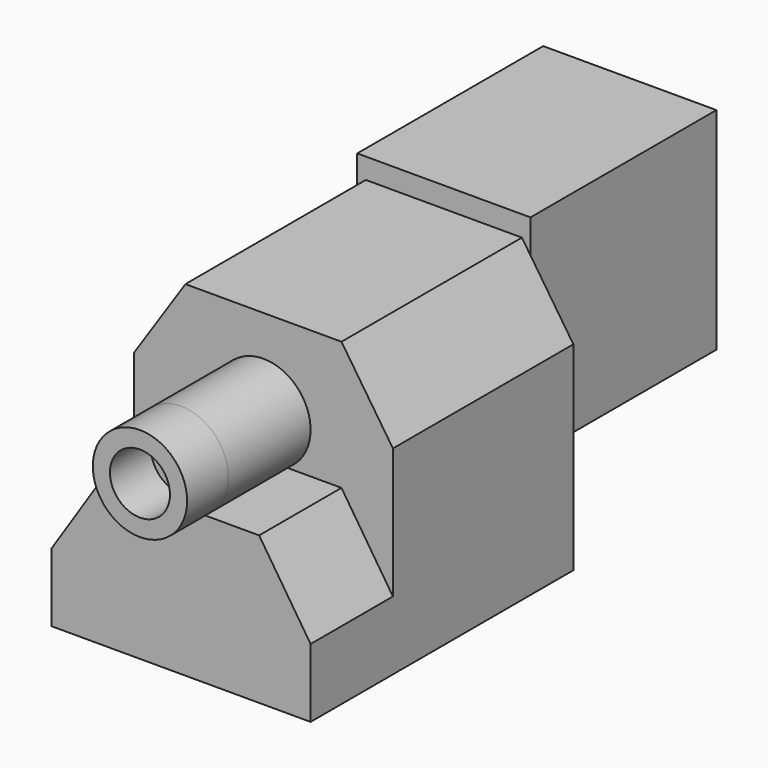
from build123d import *
from build123d import SkipClean  # not in build123d's __all__

# Parameters (mm, degrees)
F1_DEPTH = 19.15
F2_R     = 2.75
F2_R_2   = 1.75
F3_DEPTH = 3
F5_DEPTH = 6
F6_W     = 10.1
F6_H     = 12.3
F7_DEPTH = 13.55


# Not quite as in the source:
# - after a boolean that leaves OpenCascade's solid faulty, fix() repairs it


with BuildPart() as f1:
    # F0 (on Front) → F1 (new body)
    with BuildSketch(Plane.XZ):
        Polygon((4.55, 8.05), (-4.55, 8.05), (-7.55, 3.55), (-7.55, -8.05), (7.55, -8.05), (7.55, 3.55), align=None)
    extrude(amount=F1_DEPTH)

    # F2 (on face) → F3 (join)
    with BuildSketch(Plane.XZ.offset(19.15)):
        with Locations((0, 2.95)):
            Circle(F2_R)
        with Locations((0, 2.95)):
            Circle(F2_R_2, mode=Mode.SUBTRACT)
    extrude(amount=F3_DEPTH)

    # F4 (on face) → F5 (cut)
    with BuildSketch(Plane.XZ.offset(19.15)):
        with BuildLine():
            Line((-7.55, -4.05), (-4.55, 0.5498131504))
            Line((-4.55, 0.5498131504), (-1.3422380888, 0.5498131504))
            ThreePointArc((-1.3422380888, 0.5498131504), (0, 5.7), (1.3422380888, 0.5498131504))
            Line((1.3422380888, 0.5498131504), (4.55, 0.5498131504))
            Line((4.55, 0.5498131504), (7.55, -4.05))
            Line((7.55, -4.05), (7.55, 3.55))
            Line((7.55, 3.55), (4.55, 8.05))
            Line((4.55, 8.05), (-4.55, 8.05))
            Line((-4.55, 8.05), (-7.55, 3.55))
            Line((-7.55, 3.55), (-7.55, -4.05))
        make_face()
    with SkipClean():  # cleaning this boolean's faces spoils the solid; the shape is the same uncleaned
        extrude(amount=-F5_DEPTH, mode=Mode.SUBTRACT)

    # F6 (on face) → F7 (join)
    with BuildSketch(Plane(origin=(0, 0, 0), x_dir=(-1, 0, 0), z_dir=(0, 1, 0))):
        with Locations((0, 3.1)):
            Rectangle(F6_W, F6_H)
    extrude(amount=F7_DEPTH)

    add(f1.part.fix(), mode=Mode.REPLACE)


solid = f1.part
